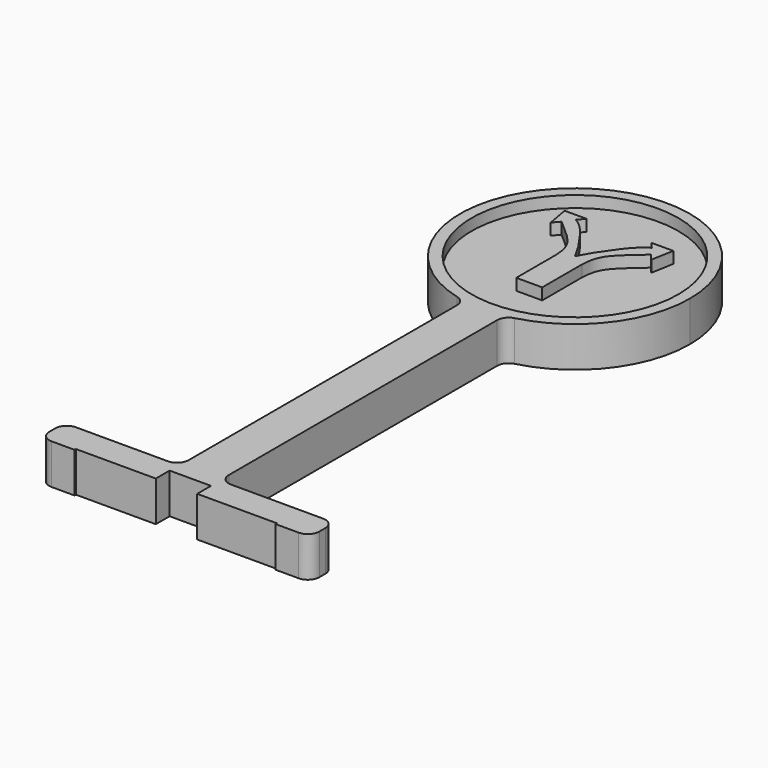
from build123d import *

# Parameters (mm, degrees)
F0_W     = 6
F0_H     = 0.3
F1_DEPTH = 7
F2_R     = 18
F3_DEPTH = 2
F4_R     = 2


# Not quite as in the source:
# - a feature names something its author has since deleted; it is built from what else it names


with BuildPart() as f1:
    # F0 (on Top) → F1 (new body)
    with BuildSketch(Plane.XY):
        with BuildLine():
            ThreePointArc((3.5, -3), (0, -3.3086313325), (-3.5, -3))
            Line((-3.5, -3), (-3.5, -65))
            Line((-3.5, -65), (-23.5, -65))
            Line((-23.5, -65), (-23.5, -70))
            Line((-23.5, -70), (-17.5, -70))
            Line((-17.5, -70), (-3.6, -70))
            Line((-3.6, -70), (-3.6, -67))
            Line((-3.6, -67), (3.6, -67))
            Line((3.6, -67), (3.6, -70))
            Line((3.6, -70), (17.5, -70))
            Line((17.5, -70), (23.5, -70))
            Line((23.5, -70), (23.5, -65))
            Line((23.5, -65), (3.5, -65))
            Line((3.5, -65), (3.5, -3))
        make_face()
        with BuildLine():
            ThreePointArc((20, 16.6913686675), (-12.8452325787, 32.0210783843), (-3.5, -3))
            ThreePointArc((-3.5, -3), (0, -3.3086313325), (3.5, -3))
            ThreePointArc((3.5, -3), (15.3297097168, 3.8461360889), (20, 16.6913686675))
        make_face()
        with Locations((-20.5, -70.15)):
            Rectangle(F0_W, F0_H)
        with Locations((20.5, -70.15)):
            Rectangle(F0_W, F0_H)
    extrude(amount=F1_DEPTH)

    # F2 (on face) → F3 (cut)
    with BuildSketch(Plane.XY.offset(7)):
        with Locations((0, 16.6913686675)):
            Circle(F2_R)
        with BuildLine():
            Line((0, 6.7382790148), (-2.256068401, 6.7382790148))
            Line((-2.256068401, 6.7382790148), (-2.256068401, 15.3757622465))
            add(Edge.make_bspline(
                [(-2.256068401, 15.3757622465), (-2.3233316964, 16.8329796939), (-2.719622442, 19.6479913649), (-7.1642837958, 22.803266535), (-7.7653425934, 23.4845241077)],
                knots=[0, 0, 0, 0, 0.4646113757, 1, 1, 1, 1], degree=3))
            Line((-7.7653425934, 23.4845241077), (-8.7472228794, 22.3505439034))
            Line((-8.7472228794, 22.3505439034), (-9.4585691677, 26.2563616887))
            Line((-9.4585691677, 26.2563616887), (-5.635671728, 26.2563616887))
            Line((-5.635671728, 26.2563616887), (-6.6175520141, 25.1223814843))
            add(Edge.make_bspline(
                [(0, 16.6913686675), (-0.8485280711, 18.3885709355), (-2.8253206301, 21.3582120071), (-5.1400469891, 24.3331446203), (-6.6175520141, 25.1223814843)],
                knots=[0, 0, 0, 0, 0.5076375045, 1, 1, 1, 1], degree=3))
            add(Edge.make_bspline(
                [(0, 16.6913686675), (0.8485280711, 18.3885709355), (2.8253206301, 21.3582120071), (5.1400469891, 24.3331446203), (6.6175520141, 25.1223814843)],
                knots=[0, 0, 0, 0, 0.5076375045, 1, 1, 1, 1], degree=3))
            Line((6.6175520141, 25.1223814843), (5.635671728, 26.2563616887))
            Line((5.635671728, 26.2563616887), (9.4585691677, 26.2563616887))
            Line((9.4585691677, 26.2563616887), (8.7472228794, 22.3505439034))
            Line((8.7472228794, 22.3505439034), (7.7653425934, 23.4845241077))
            add(Edge.make_bspline(
                [(2.256068401, 15.3757622465), (2.3233316964, 16.8329796939), (2.719622442, 19.6479913649), (7.1642837958, 22.803266535), (7.7653425934, 23.4845241077)],
                knots=[0, 0, 0, 0, 0.4646113757, 1, 1, 1, 1], degree=3))
            Line((2.256068401, 15.3757622465), (2.256068401, 6.7382790148))
            Line((2.256068401, 6.7382790148), (0, 6.7382790148))
        make_face(mode=Mode.SUBTRACT)
    extrude(amount=-F3_DEPTH, mode=Mode.SUBTRACT)

    # F4
    f4_edges = [f1.edges().sort_by_distance(p)[0] for p in [
        (-3.5, -3, 3.5),
        (3.5, -3, 3.5),
        (23.5, -65, 3.5),
        (-23.5, -65, 3.5),
        (-3.5, -65, 3.5),
        (3.5, -65, 3.5),
        (-23.5, -70.3, 3.5),
        (23.5, -70.3, 3.5),
    ]]
    fillet(f4_edges, radius=F4_R)


solid = f1.part
